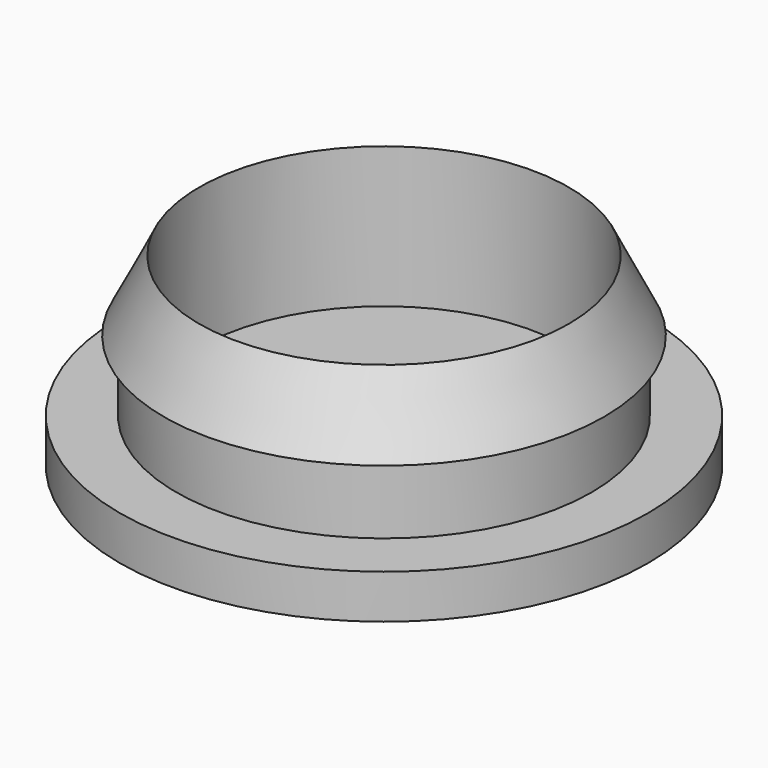
from build123d import *

# Parameters (mm, degrees)
F0_R     = 19.05
F1_DEPTH = 3.175
F2_R     = 14.986
F3_DEPTH = 5.08
F4_R     = 15.875
F5_DEPTH = 5.08
F6_SIZE2 = 5.07999
F6_SIZE  = 2.53999
F7_DEPTH = 10.16


# Not quite as in the source:
# - a fillet or chamfer is up to 0.001 mm smaller than in the source, because OpenCascade refuses the exact size


with BuildPart() as f1:
    # F0 (on Top) → F1 (new body)
    with BuildSketch(Plane.XY):
        Circle(F0_R)
    extrude(amount=F1_DEPTH)

    # F2 (on face) → F3 (join)
    with BuildSketch(Plane.XY.offset(3.175)):
        Circle(F2_R)
    extrude(amount=F3_DEPTH)

    # F4 (on face) → F5 (join)
    with BuildSketch(Plane.XY.offset(8.255)):
        Circle(F4_R)
    extrude(amount=F5_DEPTH)

    # F6 (size 2.54 and 5.08 in the source; OpenCascade refuses exactly that, so slightly less here)
    f6_edges = [f1.edges().sort_by_distance(p)[0] for p in [
        (-15.875, 0, 13.335),
    ]]
    f6_side = f1.faces().sort_by_distance((0, 0, 13.335))[0]
    chamfer(f6_edges, length=F6_SIZE, length2=F6_SIZE2, reference=f6_side)

    # F7 (cut): a face of the model
    f7_faces = [f1.faces().sort_by_distance(p)[0] for p in [
        (0, 0, 13.335),
    ]]
    extrude(f7_faces, amount=-F7_DEPTH, mode=Mode.SUBTRACT)


solid = f1.part
